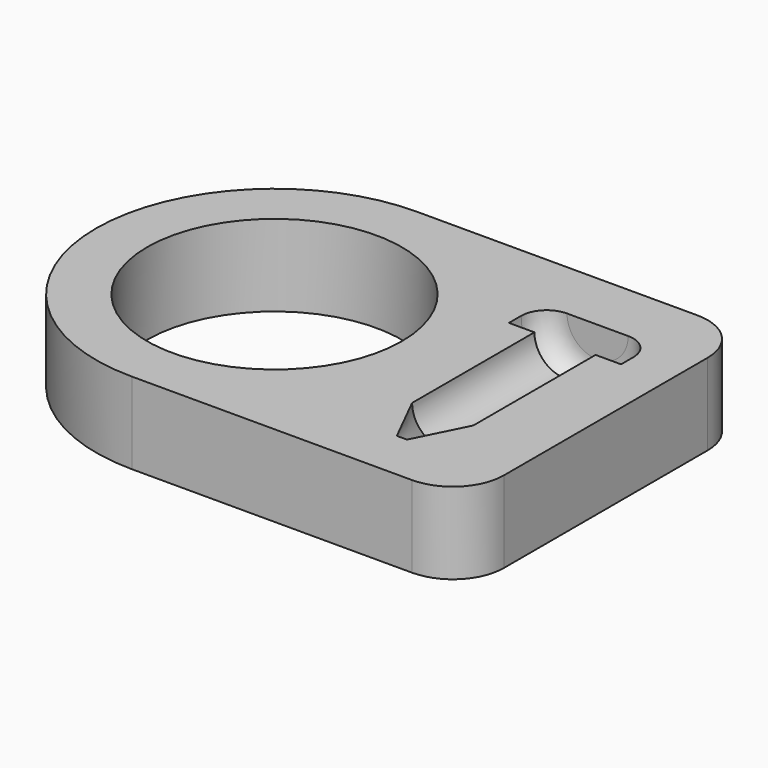
from build123d import *

# Parameters (mm, degrees)
F0_R         = 12.5
F1_DEPTH     = 8
F4_TEXT_SIZE = 5.5555555556
F5_DEPTH     = 1


# Not quite as in the source:
# - Text() gives the source's letters only with a copy of the font that has no kerning and outlines rounded to 1/6400 em; it was checked with that copy


with BuildPart() as f1:
    # F0 (on Top) → F1 (new body)
    with BuildSketch(Plane.XY):
        with BuildLine():
            ThreePointArc((0, 17.5), (5.1256313292, 5.1256313292), (17.5, 0))
            Line((17.5, 0), (45, 0))
            ThreePointArc((45, 0), (48.5355339059, 1.4644660941), (50, 5))
            Line((50, 5), (50, 30))
            ThreePointArc((50, 30), (48.5355339059, 33.5355339059), (45, 35))
            Line((45, 35), (17.5, 35))
            ThreePointArc((17.5, 35), (5.1256313292, 29.8743686708), (0, 17.5))
        make_face()
        with Locations((17.5, 17.5)):
            Circle(F0_R, mode=Mode.SUBTRACT)
    extrude(amount=F1_DEPTH)

    # F2 (on face) → F3 (revolve, cut)
    with BuildSketch(Plane.XY.offset(8)):
        with BuildLine():
            Line((40, 25), (40, 5))
            Line((40, 5), (40.5, 5))
            Line((40.5, 5), (43, 10))
            Line((43, 10), (43, 25))
            Line((43, 25), (45.5, 25))
            Line((45.5, 25), (45.5, 26.5))
            ThreePointArc((45.5, 26.5), (44.767766953, 28.267766953), (43, 29))
            Line((43, 29), (40, 29))
            Line((40, 29), (40, 25))
        make_face()
    revolve(axis=Axis((40, 15, 8), (0, 1, 0)), mode=Mode.SUBTRACT)

    # F4 (on face) → F5 (cut)
    with BuildSketch(Plane(origin=(0, 0, 0), x_dir=(1, 0, 0), z_dir=(0, 0, -1))):
        with Locations((30, -9)):
            Text('795', F4_TEXT_SIZE, font='Open Sans', text_align=(TextAlign.LEFT, TextAlign.BOTTOM))
    extrude(amount=-F5_DEPTH, mode=Mode.SUBTRACT)


solid = f1.part
